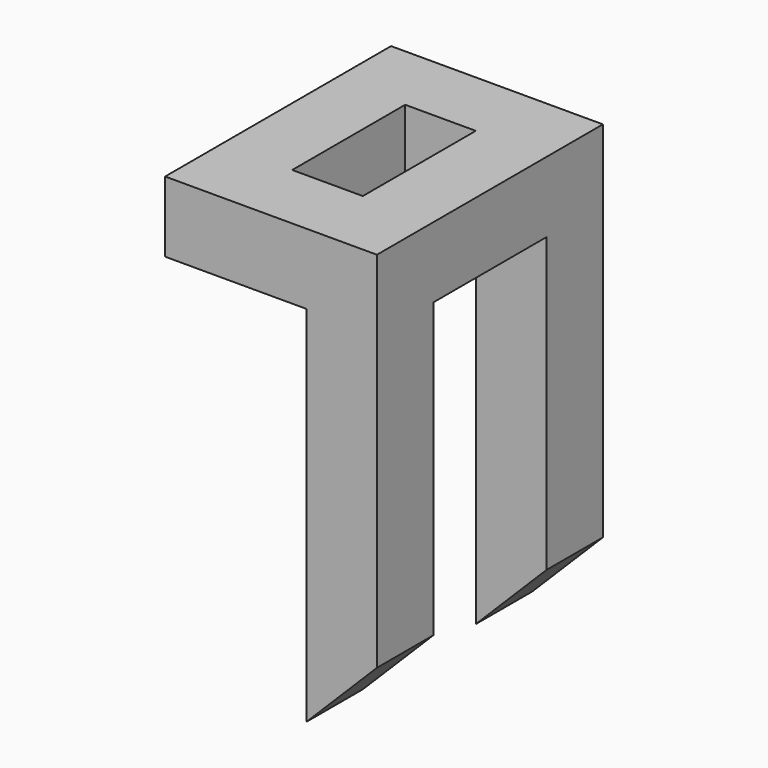
from build123d import *

# Parameters (mm, degrees)
F0_W        = 101.6
F0_H        = 25.4
F1_DEPTH    = 25.4
F2_W        = 25.4
F2_H        = 25.4
F3_DEPTH    = 25.4
F4_W        = 76.2
F4_H        = 25.4
F4_W_2      = 25.4
F5_DEPTH    = 25.4
F6_W        = 25.4
F6_H        = 25.4
F7_DEPTH    = 156.21
F8_T1_DEPTH = 286.6829915773
F8_T3_DEPTH = 286.6829915773


# Not quite as in the source:
# - a fillet or chamfer that OpenCascade refuses, or shapes differently, is made with other operations: its cross-section is extruded or revolved along the edge and cut away or added


with BuildPart() as f1:
    # F0 (on Right) → F1 (new body)
    with BuildSketch(Plane.YZ):
        Rectangle(F0_W, F0_H)
    extrude(amount=F1_DEPTH)

    # F2 (on face) → F3 (join)
    with BuildSketch(Plane.YZ.offset(25.4)):
        with Locations((38.1, 0)):
            Rectangle(F2_W, F2_H)
        with Locations((-38.1, 0)):
            Rectangle(F2_W, F2_H)
    extrude(amount=F3_DEPTH)

    # F4 (on face) → F5 (join)
    with BuildSketch(Plane.YZ.offset(50.8)):
        with Locations((12.7, 0)):
            Rectangle(F4_W, F4_H)
        with Locations((-38.1, 0)):
            Rectangle(F4_W_2, F4_H)
    extrude(amount=F5_DEPTH)

    # F6 (on face) → F7 (join)
    with BuildSketch(Plane(origin=(0, 0, -12.7), x_dir=(1, 0, 0), z_dir=(0, 0, -1))):
        with Locations((63.5, 38.1)):
            Rectangle(F6_W, F6_H)
        with Locations((63.5, -38.1)):
            Rectangle(F6_W, F6_H)
    extrude(amount=F7_DEPTH)

    # F8: chamfer of 50.8 on 2 edges, made by hand

    # F8_s2 → F8_t1 (cut)
    with BuildSketch(Plane.XZ.offset(-181.4414957887)):
        Polygon((76.2, -118.11), (25.4, -168.91), (76.2, -168.91), align=None)
    extrude(amount=F8_T1_DEPTH, mode=Mode.SUBTRACT)

    # F8_s4 → F8_t3 (cut)
    with BuildSketch(Plane.XZ.offset(-105.2414957887)):
        Polygon((25.4, -168.91), (76.2, -118.11), (76.2, -168.91), align=None)
    extrude(amount=F8_T3_DEPTH, mode=Mode.SUBTRACT)


solid = f1.part
